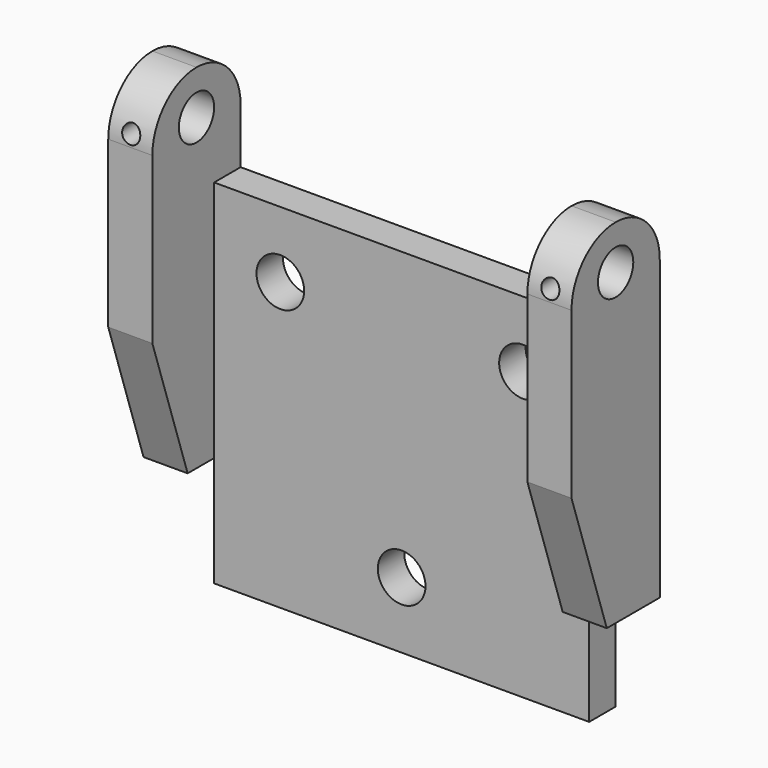
from build123d import *

# Parameters (mm, degrees)
F0_W         = 53.975
F0_H         = 50.8
F0_R         = 3.429
F1_DEPTH     = 4.7625
F2_W         = 6.35
F2_H         = 50.8
F3_DEPTH     = 15.875
F4_R         = 3.175
F5_DEPTH     = 6.35
F6_R         = 3.175
F7_DEPTH     = 6.35
F9_D         = 2.5781
F9_DEPTH     = 7.9375
F9_TIP       = 0.774539381
F10_T1_DEPTH = 46.0375
F10_T3_DEPTH = 46.0375
F11_SIZE2    = 19.05
F11_SIZE     = 6.35
F12_SIZE2    = 19.05
F12_SIZE     = 6.35


# Not quite as in the source:
# - a fillet or chamfer that OpenCascade refuses, or shapes differently, is made with other operations: its cross-section is extruded or revolved along the edge and cut away or added


with BuildPart() as f1:
    # F0 (on Front) → F1 (new body)
    with BuildSketch(Plane.XZ):
        with Locations((26.9875, 25.4)):
            Rectangle(F0_W, F0_H)
        with Locations((26.9875, 9.525)):
            Circle(F0_R, mode=Mode.SUBTRACT)
        with Locations((9.525, 41.275)):
            Circle(F0_R, mode=Mode.SUBTRACT)
        with Locations((44.45, 41.275)):
            Circle(F0_R, mode=Mode.SUBTRACT)
    extrude(amount=F1_DEPTH)

    # F2 (on Front) → F3 (join)
    with BuildSketch(Plane.XZ):
        with Locations((-3.175, 41.275)):
            Rectangle(F2_W, F2_H)
        with Locations((57.15, 41.275)):
            Rectangle(F2_W, F2_H)
    extrude(amount=F3_DEPTH)

    # F4 (on Right) → F5 (cut, through all)
    with BuildSketch(Plane.YZ):
        with Locations((-7.9375, 60.325)):
            Circle(F4_R)
    extrude(amount=-F5_DEPTH, mode=Mode.SUBTRACT)

    # F6 (on face) → F7 (cut)
    with BuildSketch(Plane.YZ.offset(60.325)):
        with Locations((-7.9375, 60.325)):
            Circle(F6_R)
    extrude(amount=-F7_DEPTH, mode=Mode.SUBTRACT)

    # F9
    with Locations(Plane.XZ.offset(15.875)):
        with Locations((-3.175, 60.325), (57.15, 60.325)):
            Hole(F9_D / 2, depth=F9_DEPTH)
            with Locations((0, 0, -(F9_DEPTH + F9_TIP / 2))):  # 118° drill point
                Cone(0, F9_D / 2, F9_TIP, mode=Mode.SUBTRACT)

    # F10: fillet of radius 7.9375 on 4 edges, made by hand

    # F10_s2 → F10_t1 (cut)
    with BuildSketch(Plane.YZ.offset(34.13125)):
        with BuildLine():
            ThreePointArc((-7.9375, 66.675), (-13.5501600757, 64.3501600757), (-15.875, 58.7375))
            Line((-15.875, 58.7375), (-15.875, 66.675))
            Line((-15.875, 66.675), (-7.9375, 66.675))
        make_face()
        with BuildLine():
            ThreePointArc((0, 58.7375), (-2.3248399243, 64.3501600757), (-7.9375, 66.675))
            Line((-7.9375, 66.675), (0, 66.675))
            Line((0, 66.675), (0, 58.7375))
        make_face()
    extrude(amount=F10_T1_DEPTH, mode=Mode.SUBTRACT)

    # F10_s4 → F10_t3 (cut)
    with BuildSketch(Plane.YZ.offset(-26.19375)):
        with BuildLine():
            ThreePointArc((-7.9375, 66.675), (-13.5501600757, 64.3501600757), (-15.875, 58.7375))
            Line((-15.875, 58.7375), (-15.875, 66.675))
            Line((-15.875, 66.675), (-7.9375, 66.675))
        make_face()
        with BuildLine():
            ThreePointArc((0, 58.7375), (-2.3248399243, 64.3501600757), (-7.9375, 66.675))
            Line((-7.9375, 66.675), (0, 66.675))
            Line((0, 66.675), (0, 58.7375))
        make_face()
    extrude(amount=F10_T3_DEPTH, mode=Mode.SUBTRACT)

    # F11
    f11_edges = [f1.edges().sort_by_distance(p)[0] for p in [
        (-3.175, -15.875, 15.875),
    ]]
    f11_side = f1.faces().sort_by_distance((-3.175, -7.9375, 15.875))[0]
    chamfer(f11_edges, length=F11_SIZE, length2=F11_SIZE2, reference=f11_side)

    # F12
    f12_edges = [f1.edges().sort_by_distance(p)[0] for p in [
        (57.15, -15.875, 15.875),
    ]]
    f12_side = f1.faces().sort_by_distance((57.15, -7.9375, 15.875))[0]
    chamfer(f12_edges, length=F12_SIZE, length2=F12_SIZE2, reference=f12_side)


solid = f1.part
